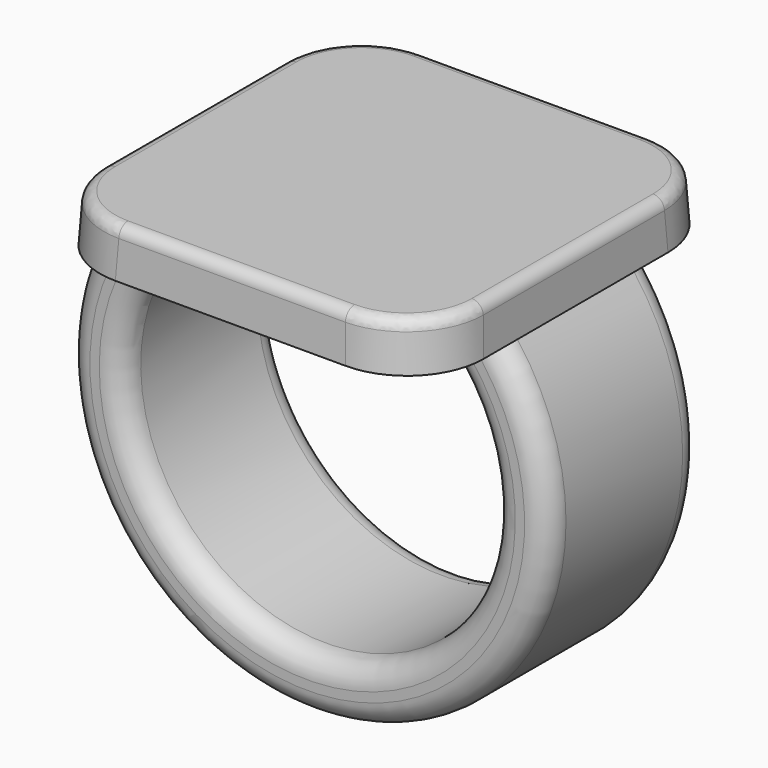
from build123d import *

# Parameters (mm, degrees)
F0_W          = 25.4
F0_H          = 25.4
F1_DEPTH      = 3.175
F1_TAPER      = 3
F3_W          = 5.08
F3_H          = 12.7
F6_DEPTH      = 6.35
F6_DEPTH_BACK = 6.35
F7_R          = 5.08
F8_R          = 1.524
F9_R          = 0.762


with BuildPart() as f1:
    # F0 (on Top) → F1 (new body)
    with BuildSketch(Plane.XY):
        Rectangle(F0_W, F0_H)
    extrude(amount=F1_DEPTH, taper=F1_TAPER)

    # F4: sweep along a path in F2
    with BuildLine(Plane.XZ) as f4_path:
        ThreePointArc((-10.16, 0), (0, -23.5582897328), (10.16, 0))
    # F3 (on face) → F4 (sweep)
    with BuildSketch(Plane(origin=(0, 0, 0), x_dir=(1, 0, 0), z_dir=(0, 0, -1))):
        with Locations((10.16, 0)):
            Rectangle(F3_W, F3_H)
    sweep(path=f4_path.line)

    # F5 (on Front) → F6 (join, two sides)
    with BuildSketch(Plane.XZ) as f6_sk:
        with BuildLine():
            Line((-7.62, 0), (-10.16, 0))
            Line((-10.16, 0), (-10.0130578512, -2.535746045))
            ThreePointArc((-10.0130578512, -2.535746045), (-8.9072265211, -1.1822790439), (-7.62, 0))
        make_face()
    extrude(amount=F6_DEPTH)
    extrude(f6_sk.sketch, amount=-F6_DEPTH_BACK)

    # F7
    f7_edges = [f1.edges().sort_by_distance(p)[0] for p in [
        (12.616803, 12.616803, 1.5875),
        (-12.616803, 12.616803, 1.5875),
        (12.616803, -12.616803, 1.5875),
        (-12.616803, -12.616803, 1.5875),
    ]]
    fillet(f7_edges, radius=F7_R)

    # F8
    f8_edges = [f1.edges().sort_by_distance(p)[0] for p in [
        (0, -6.35, -21.835726),
        (0, 6.35, -21.835726),
        (0, 6.35, -25.501344),
        (0, -6.35, -25.501344),
    ]]
    fillet(f8_edges, radius=F8_R)

    # F9
    f9_edges = [f1.edges().sort_by_distance(p)[0] for p in [
        (0, 12.533605, 3.175),
        (11.048589, 11.048589, 3.175),
        (-11.048589, 11.048589, 3.175),
        (12.533605, 0, 3.175),
        (-12.533605, 0, 3.175),
        (11.048589, -11.048589, 3.175),
        (-11.048589, -11.048589, 3.175),
        (0, -12.533605, 3.175),
    ]]
    fillet(f9_edges, radius=F9_R)


solid = f1.part
